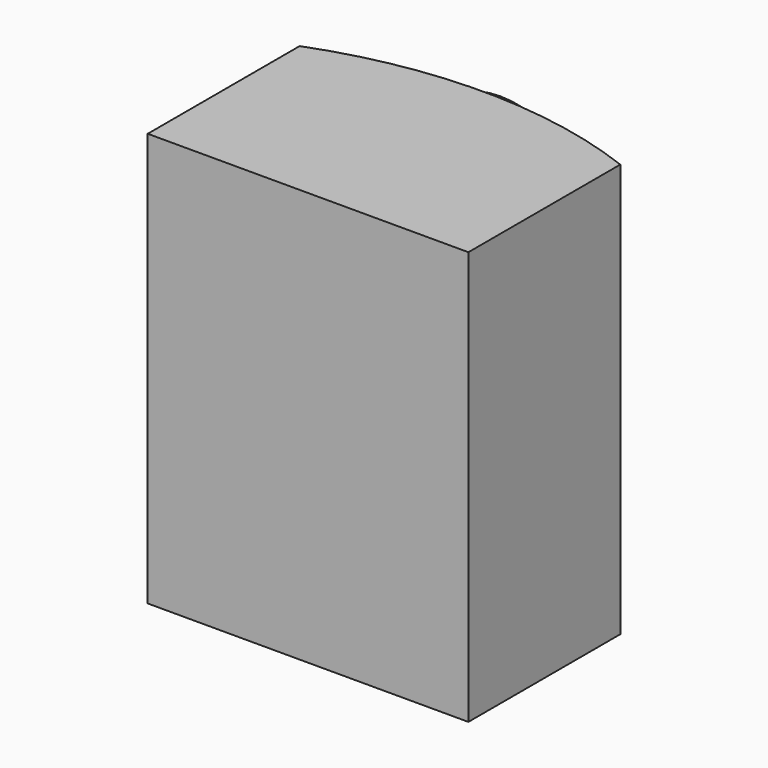
from build123d import *

# Parameters (mm, degrees)
F0_W     = 241.3
F0_H     = 311.15
F1_DEPTH = 130.175
F3_DEPTH = 311.15
F5_DEPTH = 50.8


# Not quite as in the source:
# - a length typed as a fraction of an inch, garbled in the dataset ("3 / 203.2 mm" for 3/8 in), is restored


with BuildPart() as f1:
    # F0 (on Front) → F1 (new body)
    with BuildSketch(Plane.XZ):
        Rectangle(F0_W, F0_H)
    extrude(amount=F1_DEPTH)

    # F2 (on face) → F3 (join, through all)
    with BuildSketch(Plane.XY.offset(155.575)):
        with BuildLine():
            Line((-120.65, 12.7), (-120.65, 0))
            Line((-120.65, 0), (120.65, 0))
            Line((120.65, 0), (120.65, 12.7))
            ThreePointArc((120.65, 12.7), (0, 34.925), (-120.65, 12.7))
        make_face()
    extrude(amount=-F3_DEPTH)

    # F4 (on Front) → F5 (join)
    with BuildSketch(Plane.XZ):
        with BuildLine():
            Line((69.85, 36.5125), (69.85, 76.2))
            ThreePointArc((69.85, 76.2), (0, 146.05), (-69.85, 76.2))
            Line((-69.85, 76.2), (-69.85, 36.5125))
            ThreePointArc((-69.85, 36.5125), (-33.3375, 0), (-69.85, -36.5125))
            Line((-69.85, -36.5125), (-69.85, -76.2))
            ThreePointArc((-69.85, -76.2), (0, -146.05), (69.85, -76.2))
            Line((69.85, -76.2), (69.85, -36.5125))
            ThreePointArc((69.85, -36.5125), (33.3375, 0), (69.85, 36.5125))
        make_face()
    extrude(amount=-F5_DEPTH)


solid = f1.part
